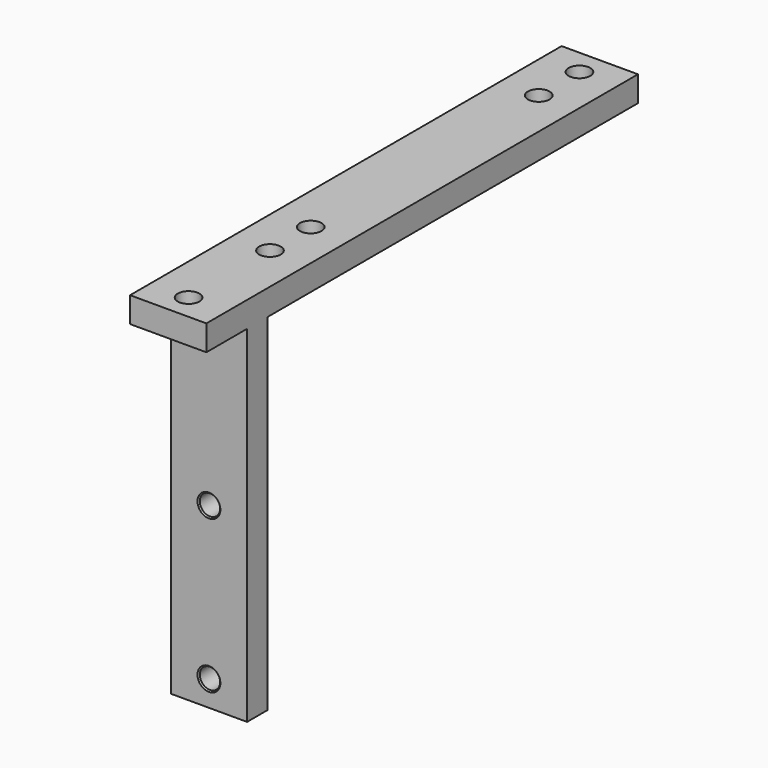
from build123d import *

# Parameters (mm, degrees)
F1_DEPTH = 30
F2_R     = 4
F3_DEPTH = 30.001
F4_SIZE  = 0.5
F5_R     = 4.25
F6_DEPTH = 146.001


with BuildPart() as f1:
    # F0 (on Right) → F1 (new body)
    with BuildSketch(Plane.YZ):
        Polygon((10, 0), (10, 136), (192, 136), (192, 146), (0, 146), (-20, 146), (-20, 136), (0, 136), (0, 0), align=None)
    extrude(amount=F1_DEPTH)

    # F2 (on face) → F3 (cut, through all)
    with BuildSketch(Plane(origin=(0, 10, 0), x_dir=(-1, 0, 0), z_dir=(0, 1, 0))):
        with Locations((-15, 70)):
            Circle(F2_R)
        with Locations((-15, 10)):
            Circle(F2_R)
    extrude(amount=-F3_DEPTH, mode=Mode.SUBTRACT)

    # F4
    f4_edges = [f1.edges().sort_by_distance(p)[0] for p in [
        (19, 10, 70),
        (11, 5, 70),
        (19, 0, 70),
        (19, 10, 10),
        (11, 5, 10),
        (19, 0, 10),
    ]]
    chamfer(f4_edges, length=F4_SIZE)

    # F5 (on face) → F6 (cut, through all)
    with BuildSketch(Plane.XY.offset(146)):
        with Locations((15, 182)):
            Circle(F5_R)
        with Locations((15, 162)):
            Circle(F5_R)
        with Locations((15, -10)):
            Circle(F5_R)
        with Locations((15, 30)):
            Circle(F5_R)
        with Locations((15, 50)):
            Circle(F5_R)
    extrude(amount=-F6_DEPTH, mode=Mode.SUBTRACT)


solid = f1.part
